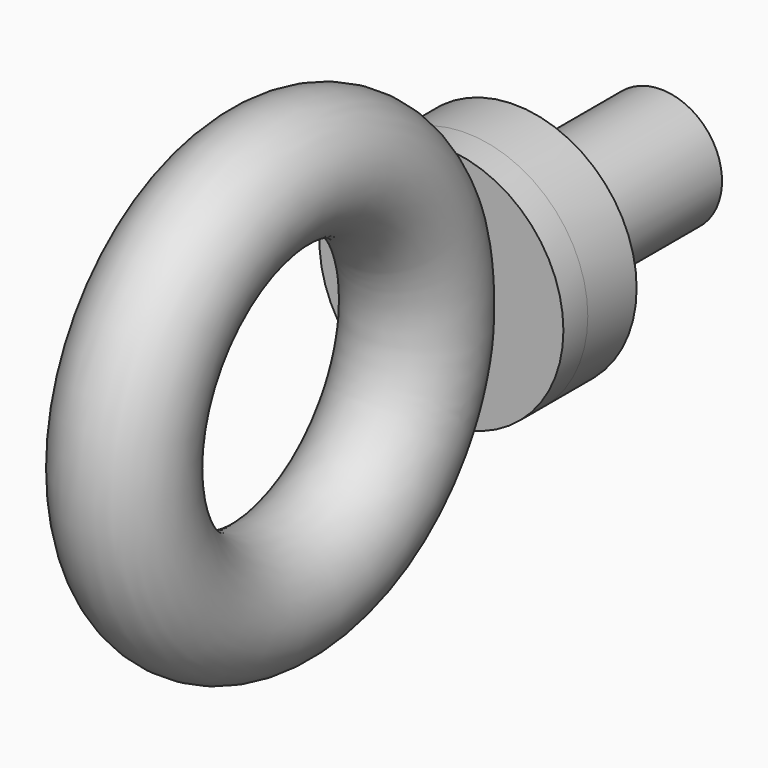
from build123d import *
from build123d import SkipClean  # not in build123d's __all__

# Parameters (mm, degrees)
F2_R     = 6.35
F3_DEPTH = 3.175
F4_R     = 3.175
F5_DEPTH = 9.525
F6_R     = 3.175
F8_DEPTH = 1.5875


with BuildPart() as f3:
    # F2 (on offset) → F3 (new body)
    with BuildSketch(Plane.XZ.offset(-12.7)):
        Circle(F2_R)
    extrude(amount=-F3_DEPTH)

    # F4 (on face) → F5 (join)
    with BuildSketch(Plane(origin=(0, 15.875, 0), x_dir=(-1, 0, 0), z_dir=(0, 1, 0))):
        Circle(F4_R)
    extrude(amount=F5_DEPTH)

    # F6 (on Top) → F7 (revolve)
    with BuildSketch(Plane.XY):
        with Locations((0, 9.525)):
            Circle(F6_R)
    with SkipClean():  # cleaning this boolean's faces spoils the solid; the shape is the same uncleaned
        revolve(axis=Axis((4.1035506874, 0, 0), (1, 0, 0)))

    # F8 (add): a face of the model
    f8_faces = [f3.faces().sort_by_distance(p)[0] for p in [
        (0, 12.7, 0),
    ]]
    extrude(f8_faces, amount=F8_DEPTH)


solid = f3.part
